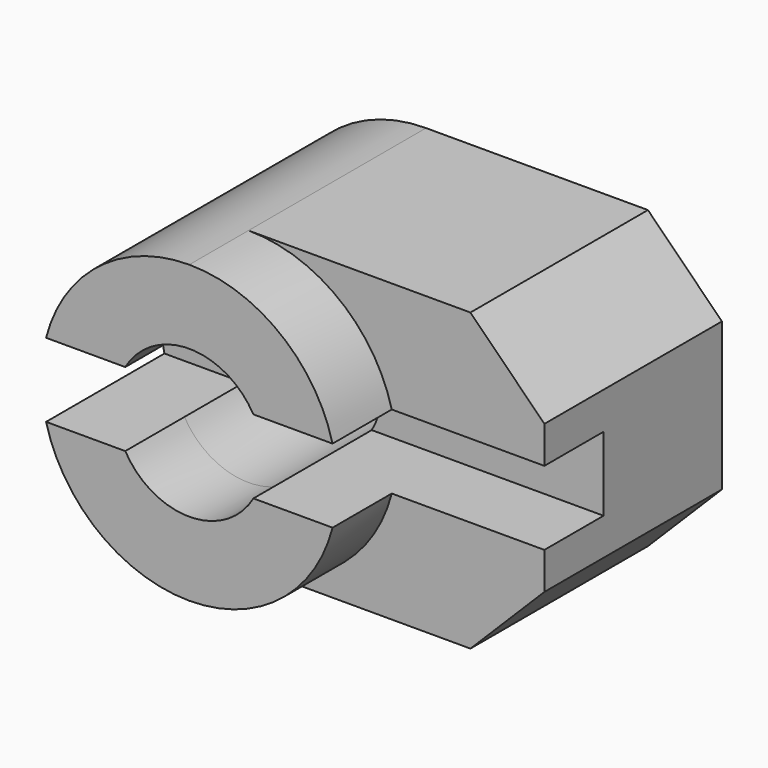
from build123d import *

# Parameters (mm, degrees)
F1_DEPTH      = 5
F2_DEPTH      = 15
F3_W          = 5
F3_H          = 5
F4_DEPTH      = 30.001
F5_R          = 5
F6_DEPTH      = 15.001
F6_DEPTH_BACK = 5.001


with BuildPart() as f1:
    # F0 (on Front) → F1 (new body)
    with BuildSketch(Plane.XZ):
        with BuildLine():
            ThreePointArc((0, -10), (7.071068, -7.071068), (10, 0))
            ThreePointArc((10, 0), (7.071068, 7.071068), (0, 10))
            ThreePointArc((0, 10), (-10, 0), (0, -10))
        make_face()
    extrude(amount=F1_DEPTH)

    # F0 (on Front) → F2 (join)
    with BuildSketch(Plane.XZ):
        with BuildLine():
            ThreePointArc((0, -10), (7.071068, -7.071068), (10, 0))
            ThreePointArc((10, 0), (7.071068, 7.071068), (0, 10))
            ThreePointArc((0, 10), (-10, 0), (0, -10))
        make_face()
        with BuildLine():
            ThreePointArc((0, 10), (7.071068, 7.071068), (10, 0))
            ThreePointArc((10, 0), (7.071068, -7.071068), (0, -10))
            Line((0, -10), (15, -10))
            Line((15, -10), (20, -5))
            Line((20, -5), (20, 5))
            Line((20, 5), (15, 10))
            Line((15, 10), (0, 10))
        make_face()
    extrude(amount=-F2_DEPTH)

    # F3 (on face) → F4 (cut, through all)
    with BuildSketch(Plane.YZ.offset(20)):
        with Locations((2.5, 0)):
            Rectangle(F3_W, F3_H)
        with Locations((-2.5, 0)):
            Rectangle(F3_W, F3_H)
    extrude(amount=-F4_DEPTH, mode=Mode.SUBTRACT)

    # F5 (on face) → F6 (cut, two sides)
    with BuildSketch(Plane.XZ) as f6_sk:
        Circle(F5_R)
    extrude(amount=-F6_DEPTH, mode=Mode.SUBTRACT)
    extrude(f6_sk.sketch, amount=F6_DEPTH_BACK, mode=Mode.SUBTRACT)


solid = f1.part
